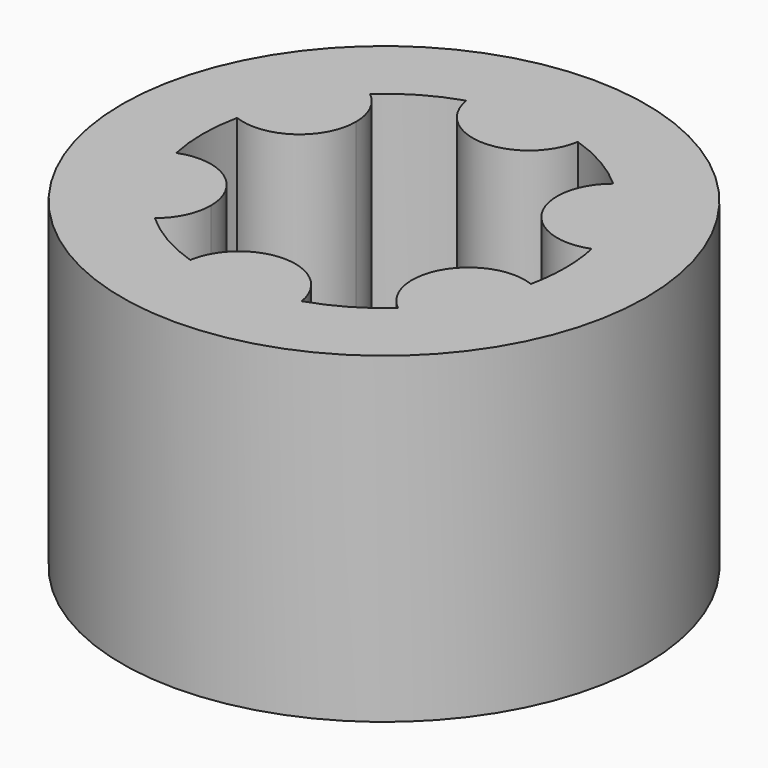
from build123d import *

# Parameters (mm, degrees)
F0_R     = 3.25
F1_DEPTH = 4


with BuildPart() as f1:
    # F0 (on Top) → F1 (new body)
    with BuildSketch(Plane.XY):
        Circle(F0_R)
        with BuildLine():
            ThreePointArc((2.1999961154, 0.4717171738), (2.2374641069, 0.2371800374), (2.25, 0))
            ThreePointArc((2.25, 0), (2.2374641069, -0.2371800374), (2.1999961154, -0.4717171738))
            ThreePointArc((2.1999961154, -0.4717171738), (2.5256218299, -0.7287723318), (2.6485571585, -1.125))
            ThreePointArc((2.6485571585, -1.125), (2.2501959894, -1.7566755621), (1.5085171137, -1.6693939373))
            ThreePointArc((1.5085171137, -1.6693939373), (1.125, -1.9485571585), (0.6914790018, -2.1411111111))
            ThreePointArc((0.6914790018, -2.1411111111), (0.6978664991, -2.1953891093), (0.7, -2.25))
            ThreePointArc((0.7, -2.25), (-0.0546108907, -2.9478664991), (-0.6914790018, -2.1411111111))
            ThreePointArc((-0.6914790018, -2.1411111111), (-1.125, -1.9485571585), (-1.5085171137, -1.6693939373))
            ThreePointArc((-1.5085171137, -1.6693939373), (-2.5547749412, -1.475), (-2.1999961154, -0.4717171738))
            ThreePointArc((-2.1999961154, -0.4717171738), (-2.25, 0), (-2.1999961154, 0.4717171738))
            ThreePointArc((-2.1999961154, 0.4717171738), (-2.5547749412, 1.475), (-1.5085171137, 1.6693939373))
            ThreePointArc((-1.5085171137, 1.6693939373), (-1.125, 1.9485571585), (-0.6914790018, 2.1411111111))
            ThreePointArc((-0.6914790018, 2.1411111111), (-0.0546108907, 2.9478664991), (0.7, 2.25))
            ThreePointArc((0.7, 2.25), (0.6978664991, 2.1953891093), (0.6914790018, 2.1411111111))
            ThreePointArc((0.6914790018, 2.1411111111), (1.125, 1.9485571585), (1.5085171137, 1.6693939373))
            ThreePointArc((1.5085171137, 1.6693939373), (2.2501959894, 1.7566755621), (2.6485571585, 1.125))
            ThreePointArc((2.6485571585, 1.125), (2.5256218299, 0.7287723318), (2.1999961154, 0.4717171738))
        make_face(mode=Mode.SUBTRACT)
        with BuildLine():
            ThreePointArc((1.5085171137, 1.6693939373), (1.9485571585, 1.125), (2.1999961154, 0.4717171738))
            ThreePointArc((2.1999961154, 0.4717171738), (2.5256218299, 0.7287723318), (2.6485571585, 1.125))
            ThreePointArc((2.6485571585, 1.125), (2.2501959894, 1.7566755621), (1.5085171137, 1.6693939373))
        make_face()
        with BuildLine():
            ThreePointArc((2.6485571585, -1.125), (2.5256218299, -0.7287723318), (2.1999961154, -0.4717171738))
            ThreePointArc((2.1999961154, -0.4717171738), (1.9485571585, -1.125), (1.5085171137, -1.6693939373))
            ThreePointArc((1.5085171137, -1.6693939373), (2.2501959894, -1.7566755621), (2.6485571585, -1.125))
        make_face()
        with BuildLine():
            ThreePointArc((-0.6914790018, 2.1411111111), (0, 2.25), (0.6914790018, 2.1411111111))
            ThreePointArc((0.6914790018, 2.1411111111), (0.6978664991, 2.1953891093), (0.7, 2.25))
            ThreePointArc((0.7, 2.25), (-0.0546108907, 2.9478664991), (-0.6914790018, 2.1411111111))
        make_face()
        with BuildLine():
            ThreePointArc((0.7, -2.25), (0.6978664991, -2.1953891093), (0.6914790018, -2.1411111111))
            ThreePointArc((0.6914790018, -2.1411111111), (0, -2.25), (-0.6914790018, -2.1411111111))
            ThreePointArc((-0.6914790018, -2.1411111111), (-0.0546108907, -2.9478664991), (0.7, -2.25))
        make_face()
        with BuildLine():
            ThreePointArc((-2.1999961154, 0.4717171738), (-1.9485571585, 1.125), (-1.5085171137, 1.6693939373))
            ThreePointArc((-1.5085171137, 1.6693939373), (-2.5547749412, 1.475), (-2.1999961154, 0.4717171738))
        make_face()
        with BuildLine():
            ThreePointArc((-2.1999961154, -0.4717171738), (-2.5547749412, -1.475), (-1.5085171137, -1.6693939373))
            ThreePointArc((-1.5085171137, -1.6693939373), (-1.9485571585, -1.125), (-2.1999961154, -0.4717171738))
        make_face()
        with BuildLine():
            ThreePointArc((1.5085171137, 1.6693939373), (1.3423393759, 0.775), (2.1999961154, 0.4717171738))
            ThreePointArc((2.1999961154, 0.4717171738), (1.9485571585, 1.125), (1.5085171137, 1.6693939373))
        make_face()
        with BuildLine():
            ThreePointArc((1.5085171137, -1.6693939373), (1.9485571585, -1.125), (2.1999961154, -0.4717171738))
            ThreePointArc((2.1999961154, -0.4717171738), (1.3423393759, -0.775), (1.5085171137, -1.6693939373))
        make_face()
        with BuildLine():
            ThreePointArc((-0.6914790018, 2.1411111111), (0, 1.55), (0.6914790018, 2.1411111111))
            ThreePointArc((0.6914790018, 2.1411111111), (0, 2.25), (-0.6914790018, 2.1411111111))
        make_face()
        with BuildLine():
            ThreePointArc((-0.6914790018, -2.1411111111), (0, -2.25), (0.6914790018, -2.1411111111))
            ThreePointArc((0.6914790018, -2.1411111111), (0, -1.55), (-0.6914790018, -2.1411111111))
        make_face()
        with BuildLine():
            ThreePointArc((-1.2485571585, 1.125), (-1.3168815965, 1.4266388309), (-1.5085171137, 1.6693939373))
            ThreePointArc((-1.5085171137, 1.6693939373), (-1.9485571585, 1.125), (-2.1999961154, 0.4717171738))
            ThreePointArc((-2.1999961154, 0.4717171738), (-1.5523294903, 0.5479353287), (-1.2485571585, 1.125))
        make_face()
        with BuildLine():
            ThreePointArc((-2.1999961154, -0.4717171738), (-1.9485571585, -1.125), (-1.5085171137, -1.6693939373))
            ThreePointArc((-1.5085171137, -1.6693939373), (-1.3168815965, -1.4266388309), (-1.2485571585, -1.125))
            ThreePointArc((-1.2485571585, -1.125), (-1.5523294903, -0.5479353287), (-2.1999961154, -0.4717171738))
        make_face()
    extrude(amount=F1_DEPTH)


solid = f1.part
